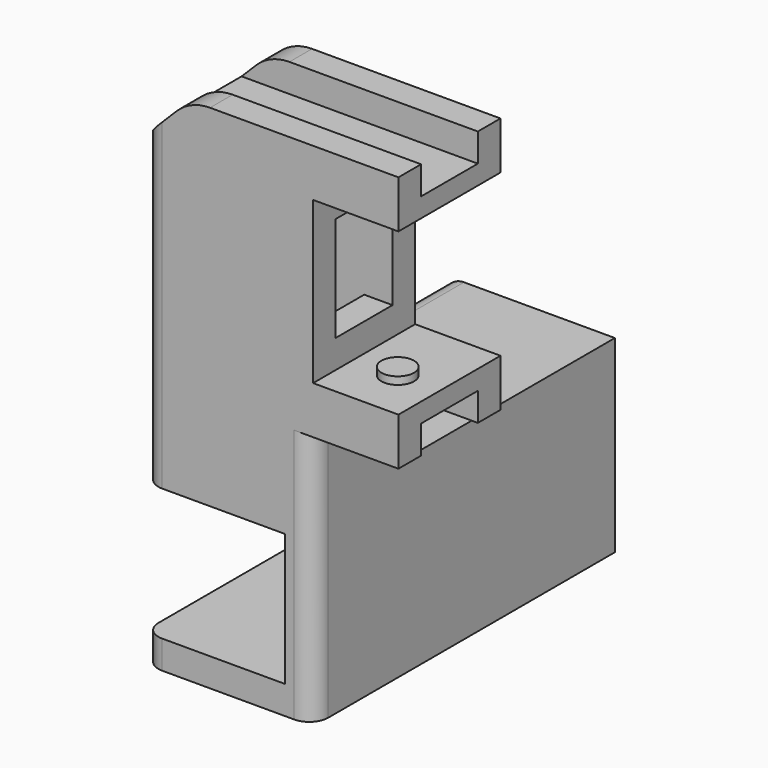
from build123d import *

# Parameters (mm, degrees)
F0_W      = 18
F0_H      = 21.2
F1_DEPTH  = 40
F2_W      = 13.525
F2_H      = 2.05
F3_DEPTH  = 9.05
F4_R      = 1.732
F5_DEPTH  = 0.8
F7_W      = 18
F7_H      = 13.525
F8_DEPTH  = 30
F9_W      = 18
F9_H      = 20
F10_DEPTH = 26.475
F11_W     = 18
F11_H     = 26.475
F12_DEPTH = 21.2
F13_W     = 15
F13_H     = 14
F14_DEPTH = 35
F16_D     = 4.5
F17_W     = 7.525
F17_H     = 28.2
F18_DEPTH = 15
F19_W     = 7.525
F19_H     = 11.1
F20_DEPTH = 18.001
F21_W     = 27.05
F21_H     = 3
F22_DEPTH = 3
F23_W     = 9.05
F23_H     = 3
F24_DEPTH = 3
F25_SIZE  = 5
F26_R     = 2
F27_R     = 5


# Not quite as in the source:
# - a pattern or mirror of a feature is missing from the dataset's text; its kind, count and spacing are read off the source's solid


with BuildPart() as f1:
    # F0 (on Front) → F1 (new body)
    with BuildSketch(Plane.XZ):
        with Locations((9, -10.6)):
            Rectangle(F0_W, F0_H)
    extrude(amount=F1_DEPTH)

    # F2 (on face) → F3 (join)
    with BuildSketch(Plane.YZ.offset(18)):
        with Locations((-33.2375, -1.025)):
            Rectangle(F2_W, F2_H)
        with Locations((-33.2375, -20.175)):
            Rectangle(F2_W, F2_H)
    extrude(amount=F3_DEPTH)

    # F4 (on face) → F5 (join)
    with BuildSketch(Plane(origin=(0, 0, -2.05), x_dir=(1, 0, 0), z_dir=(0, 0, -1))):
        with Locations((22.6, 34.5260798931)):
            Circle(F4_R)
    f5 = extrude(amount=F5_DEPTH)

    # F5_copies: F5 across plane
    add(f5.mirror(Plane(origin=(0, 0, -10.6), x_dir=(-1, 0, 0), z_dir=(0, 0, -1))))

    # F7 (on face) → F8 (join)
    with BuildSketch(Plane(origin=(0, 0, -21.2), x_dir=(1, 0, 0), z_dir=(0, 0, -1))):
        with Locations((9, 33.2375)):
            Rectangle(F7_W, F7_H)
    extrude(amount=F8_DEPTH)

    # F9 (on face) → F10 (join, through all)
    with BuildSketch(Plane(origin=(0, -26.475, 0), x_dir=(-1, 0, 0), z_dir=(0, 1, 0))):
        with Locations((-9, -41.2)):
            Rectangle(F9_W, F9_H)
    extrude(amount=F10_DEPTH)

    # F11 (on face) → F12 (cut, through all)
    with BuildSketch(Plane(origin=(0, 0, -21.2), x_dir=(1, 0, 0), z_dir=(0, 0, -1))):
        with Locations((9, 13.2375)):
            Rectangle(F11_W, F11_H)
    extrude(amount=-F12_DEPTH, mode=Mode.SUBTRACT)

    # F13 (on face) → F14 (cut)
    with BuildSketch(Plane.XZ.offset(40)):
        with Locations((7.5, -41.2)):
            Rectangle(F13_W, F13_H)
    extrude(amount=-F14_DEPTH, mode=Mode.SUBTRACT)

    # F16 (through all)
    with Locations(Plane(origin=(0, 0, 0), x_dir=(-1, 0, 0), z_dir=(0, 1, 0))):
        with Locations((-10, -41.2)):
            Hole(F16_D / 2)

    # F17 (on face) → F18 (cut)
    with BuildSketch(Plane(origin=(0, 0, 0), x_dir=(0, -1, 0), z_dir=(-1, 0, 0))):
        with Locations((33.2375, -17.1)):
            Rectangle(F17_W, F17_H)
    extrude(amount=-F18_DEPTH, mode=Mode.SUBTRACT)

    # F19 (on face) → F20 (cut, through all)
    with BuildSketch(Plane.YZ.offset(18)):
        with Locations((-33.2375, -10.6)):
            Rectangle(F19_W, F19_H)
    extrude(amount=-F20_DEPTH, mode=Mode.SUBTRACT)

    # F21 (on face) → F22 (join)
    with BuildSketch(Plane.XY):
        with Locations((13.525, -38.5)):
            Rectangle(F21_W, F21_H)
        with Locations((13.525, -27.975)):
            Rectangle(F21_W, F21_H)
    extrude(amount=F22_DEPTH)

    # F23 (on face) → F24 (join)
    with BuildSketch(Plane(origin=(0, 0, -21.2), x_dir=(1, 0, 0), z_dir=(0, 0, -1))):
        with Locations((22.525, 38.5)):
            Rectangle(F23_W, F23_H)
        with Locations((22.525, 27.975)):
            Rectangle(F23_W, F23_H)
    extrude(amount=F24_DEPTH)

    # F25
    f25_edges = [f1.edges().sort_by_distance(p)[0] for p in [
        (0, -27.975, 3),
    ]]
    chamfer(f25_edges, length=F25_SIZE)

    # F26
    f26_edges = [f1.edges().sort_by_distance(p)[0] for p in [
        (0, -40, -49.7),
        (0, -40, -18.1),
        (0, -13.2375, -31.2),
        (18, -40, -37.7),
        (0, -26.475, -16.6),
    ]]
    fillet(f26_edges, radius=F26_R)

    # F27
    f27_edges = [f1.edges().sort_by_distance(p)[0] for p in [
        (5, -38.5, 3),
        (5, -27.975, 3),
    ]]
    fillet(f27_edges, radius=F27_R)


solid = f1.part
